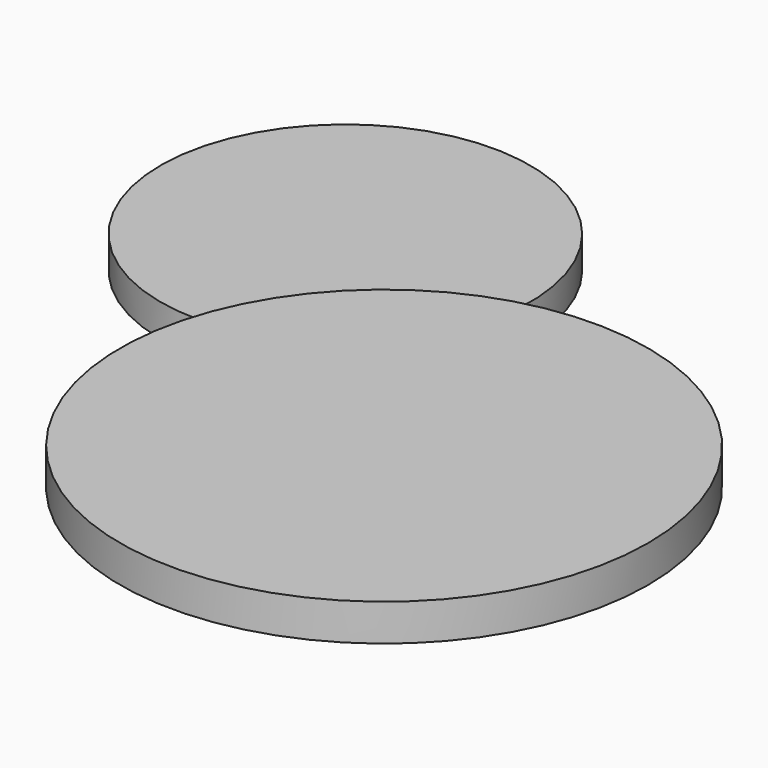
from build123d import *

# Parameters (mm, degrees)
F0_R     = 45.4264062375
F1_DEPTH = 6.35
F2_R     = 31.826020393
F3_DEPTH = 5.588


# Not quite as in the source:
# - the program builds the solid bodies; features that only make, move or delete a surface that nothing else refers to are left out


with BuildPart() as f1:
    # F0 (on Top) → F1 (new body)
    with BuildSketch(Plane.XY):
        Circle(F0_R)
    extrude(amount=F1_DEPTH)

    # F2 (on Top) → F3 (join)
    with BuildSketch(Plane.XY):
        with Locations((-43.5032360256, 46.0441485047)):
            Circle(F2_R)
    extrude(amount=F3_DEPTH)


solid = f1.part
